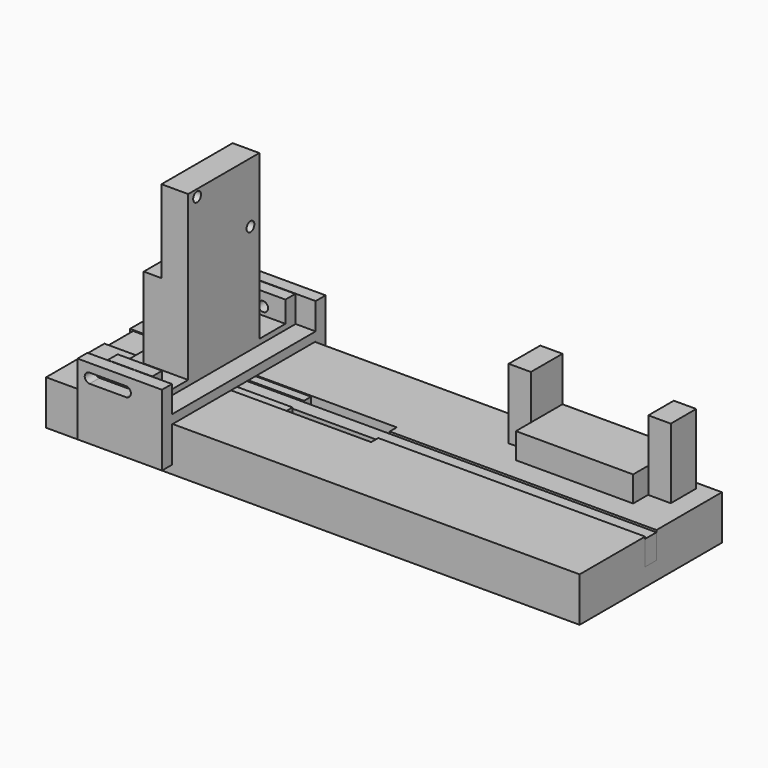
from build123d import *

# Parameters (mm, degrees)
F0_W      = 152.4
F0_H      = 50.8
F1_DEPTH  = 12.7
F2_W      = 152.4
F2_H      = 4.064
F3_DEPTH  = 7.62
F4_W      = 125.476
F4_H      = 4.0386
F5_DEPTH  = 7.0358
F6_W      = 76.2
F6_H      = 9.144
F7_DEPTH  = 7.62
F8_W      = 50.8
F8_H      = 9.1151185334
F9_DEPTH  = 7.366
F10_W     = 1.27
F10_H     = 44.45
F11_DEPTH = 25.4
F12_W     = 6.35
F12_H     = 11.2776
F12_W_2   = 6.4000114799
F12_H_2   = 9.0863150216
F13_DEPTH = 20.0152
F14_W     = 33.4765905678
F14_H     = 16.6260491401
F15_DEPTH = 7.3152
F16_W     = 25.4
F16_H     = 4.064
F17_DEPTH = 25.4
F18_R     = 1.8415
F19_DEPTH = 5.08
F20_R     = 1.0795
F21_DEPTH = 25.4
F22_W     = 24.13
F22_H     = 58.42
F23_DEPTH = 2.54
F24_W     = 24.13
F24_H     = 3.5704082614
F24_H_2   = 3.5550768292
F25_DEPTH = 10.16
F27_DEPTH = 140.208
F28_W     = 12.7008110285
F28_H     = 51.0461516678
F29_DEPTH = 7.62
F30_W     = 12.7008110285
F30_H     = 44.0202057362
F31_DEPTH = 5.08
F32_W     = 12.7008110285
F32_H     = 25.4
F33_DEPTH = 45.72
F34_R     = 1.397
F35_DEPTH = 25.4
F36_W     = 5.0705485046
F36_H     = 25.4
F37_DEPTH = 23.622
F40_DEPTH = 1.016
F38_R     = 1.4024669373
F41_DEPTH = 8.5598
F39_R     = 1.397
F42_DEPTH = 7.5438


with BuildPart() as f1:
    # F0 (on Top) → F1 (new body)
    with BuildSketch(Plane.XY):
        Rectangle(F0_W, F0_H)
    extrude(amount=F1_DEPTH)

    # F2 (on face) → F3 (cut)
    with BuildSketch(Plane.XY.offset(12.7)):
        Rectangle(F2_W, F2_H)
    extrude(amount=-F3_DEPTH, mode=Mode.SUBTRACT)

    # F6 (on face) → F7 (cut)
    with BuildSketch(Plane.XY.offset(12.7)):
        with Locations((-38.1, 0)):
            Rectangle(F6_W, F6_H)
    extrude(amount=-F7_DEPTH, mode=Mode.SUBTRACT)

    # F10 (on face) → F11 (cut)
    with BuildSketch(Plane.XY.offset(12.7)):
        with Locations((-66.4477199316, 0)):
            Rectangle(F10_W, F10_H)
    extrude(amount=-F11_DEPTH, mode=Mode.SUBTRACT)

    # F12 (on face) → F13 (join)
    with BuildSketch(Plane.XY.offset(12.7)):
        with Locations((27.48235901, 19.7612)):
            Rectangle(F12_W, F12_H)
        with Locations((67.4071349204, 18.6655575108)):
            Rectangle(F12_W_2, F12_H_2)
    extrude(amount=F13_DEPTH)

    # F14 (on face) → F15 (join)
    with BuildSketch(Plane.XY.offset(12.7)):
        with Locations((47.3956542939, 17.08697543)):
            Rectangle(F14_W, F14_H)
    extrude(amount=F15_DEPTH)


with BuildPart() as f5:
    # F4 (on face) → F5 (new body)
    with BuildSketch(Plane.XY.offset(5.08)):
        with Locations((13.4619977325, 0)):
            Rectangle(F4_W, F4_H)
    extrude(amount=F5_DEPTH)


with BuildPart() as f9:
    # F8 (on face) → F9 (new body)
    with BuildSketch(Plane.XY.offset(5.08)):
        with Locations((-49.8929896116, 0.0044535846)):
            Rectangle(F8_W, F8_H)
    extrude(amount=F9_DEPTH)

    # F16 (on face) → F17 (cut)
    with BuildSketch(Plane.XY.offset(12.446)):
        with Locations((-37.1929896116, 0)):
            Rectangle(F16_W, F16_H)
    extrude(amount=-F17_DEPTH, mode=Mode.SUBTRACT)

    # F18 (on face) → F19 (cut)
    with BuildSketch(Plane(origin=(-75.2929896116, 0, 0), x_dir=(0, -1, 0), z_dir=(-1, 0, 0))):
        with Locations((-0.0044535846, 6.9342)):
            Circle(F18_R)
    extrude(amount=-F19_DEPTH, mode=Mode.SUBTRACT)

    # F20 (on face) → F21 (cut, symmetric)
    with BuildSketch(Plane.XZ.offset(-2.032)):
        with Locations((-46.9719896116, 7.112)):
            Circle(F20_R)
        with Locations((-26.3217896116, 7.112)):
            Circle(F20_R)
    extrude(amount=F21_DEPTH, both=True, mode=Mode.SUBTRACT)


with BuildPart() as f23:
    # F22 (on face) → F23 (new body)
    with BuildSketch(Plane.XY.offset(12.7)):
        with Locations((-52.1161258221, 0)):
            Rectangle(F22_W, F22_H)
    extrude(amount=F23_DEPTH)

    # F24 (on face) → F25 (join, symmetric)
    with BuildSketch(Plane(origin=(0, 0, 12.7), x_dir=(1, 0, 0), z_dir=(0, 0, -1))):
        with Locations((-52.1161258221, 27.4247958693)):
            Rectangle(F24_W, F24_H)
        with Locations((-52.1161258221, -27.4324615854)):
            Rectangle(F24_W, F24_H_2)
    extrude(amount=F25_DEPTH, both=True)

    # F26 (on face) → F27 (cut, symmetric)
    with BuildSketch(Plane.XZ.offset(-25.6549231708)):
        with BuildLine():
            ThreePointArc((-60.7163496315, 17.653), (-59.7285214582, 18.0621718267), (-59.3193496315, 19.05))
            ThreePointArc((-59.3193496315, 19.05), (-59.7285214582, 20.0378281733), (-60.7163496315, 20.447))
            Line((-60.7163496315, 20.447), (-60.7163496315, 17.653))
        make_face()
        with BuildLine():
            ThreePointArc((-60.7163496315, 20.447), (-59.7285214582, 20.0378281733), (-59.3193496315, 19.05))
            ThreePointArc((-59.3193496315, 19.05), (-59.7285214582, 18.0621718267), (-60.7163496315, 17.653))
            Line((-60.7163496315, 17.653), (-50.3274984658, 17.653))
            ThreePointArc((-50.3274984658, 17.653), (-51.7244984658, 19.05), (-50.3274984658, 20.447))
            Line((-50.3274984658, 20.447), (-60.7163496315, 20.447))
        make_face()
        with BuildLine():
            Line((-60.7163496315, 17.653), (-60.7163496315, 20.447))
            ThreePointArc((-60.7163496315, 20.447), (-62.1133496315, 19.05), (-60.7163496315, 17.653))
        make_face()
        with BuildLine():
            Line((-50.3274984658, 17.653), (-50.3274984658, 20.447))
            ThreePointArc((-50.3274984658, 20.447), (-51.7244984658, 19.05), (-50.3274984658, 17.653))
        make_face()
        with BuildLine():
            ThreePointArc((-48.9304984658, 19.05), (-49.3396702925, 20.0378281733), (-50.3274984658, 20.447))
            Line((-50.3274984658, 20.447), (-50.3274984658, 17.653))
            ThreePointArc((-50.3274984658, 17.653), (-49.3396702925, 18.0621718267), (-48.9304984658, 19.05))
        make_face()
    extrude(amount=F27_DEPTH, both=True, mode=Mode.SUBTRACT)


with BuildPart() as f29:
    # F28 (on face) → F29 (new body)
    with BuildSketch(Plane.XY.offset(15.24)):
        with Locations((-52.1161258221, 0)):
            Rectangle(F28_W, F28_H)
    extrude(amount=F29_DEPTH)

    # F30 (on face) → F31 (cut)
    with BuildSketch(Plane.XY.offset(22.86)):
        with Locations((-52.1161258221, 0)):
            Rectangle(F30_W, F30_H)
    extrude(amount=-F31_DEPTH, mode=Mode.SUBTRACT)

    # F32 (on face) → F33 (join)
    with BuildSketch(Plane.XY.offset(17.78)):
        with Locations((-52.1161258221, 0)):
            Rectangle(F32_W, F32_H)
    extrude(amount=F33_DEPTH)

    # F34 (on face) → F35 (cut)
    with BuildSketch(Plane(origin=(-58.4665313363, 0, 0), x_dir=(0, -1, 0), z_dir=(-1, 0, 0))):
        with Locations((9.525, 61.5188)):
            Circle(F34_R)
        with Locations((-9.525, 46.2788)):
            Circle(F34_R)
    extrude(amount=-F35_DEPTH, mode=Mode.SUBTRACT)

    # F36 (on face) → F37 (cut)
    with BuildSketch(Plane.XY.offset(63.5)):
        with Locations((-55.931257084, 0)):
            Rectangle(F36_W, F36_H)
    extrude(amount=-F37_DEPTH, mode=Mode.SUBTRACT)

    # F40 (cut): faces of the model
    f40_faces = [f29.faces().sort_by_distance(p)[0] for p in [
        (-52.1161258221, 17.355051434, 17.78),
        (-52.1161258221, -17.355051434, 17.78),
    ]]
    extrude(f40_faces, amount=-F40_DEPTH, mode=Mode.SUBTRACT)

    # F38 (on face) → F41 (cut)
    with BuildSketch(Plane.XZ.offset(25.5230758339)):
        with Locations((-52.1161258221, 19.05)):
            Circle(F38_R)
    extrude(amount=-F41_DEPTH, mode=Mode.SUBTRACT)

    # F39 (on face) → F42 (cut)
    with BuildSketch(Plane(origin=(0, 25.5230758339, 0), x_dir=(-1, 0, 0), z_dir=(0, 1, 0))):
        with Locations((52.1161258221, 19.05)):
            Circle(F39_R)
    extrude(amount=-F42_DEPTH, mode=Mode.SUBTRACT)


solid = Compound([f1.part, f5.part, f9.part, f23.part, f29.part])
